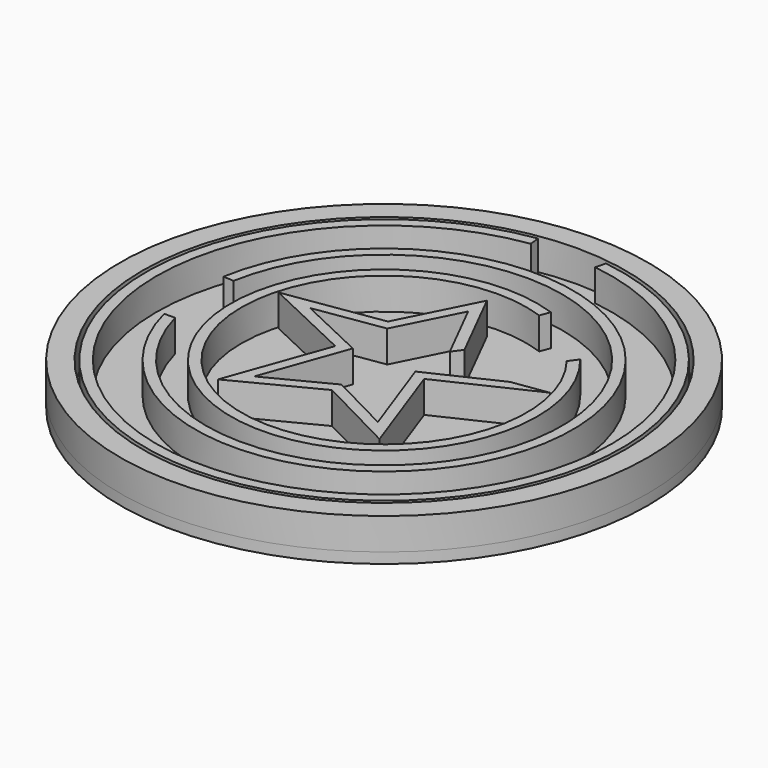
from build123d import *

# Parameters (mm, degrees)
F0_R     = 50
F0_R_2   = 45.8000004292
F1_DEPTH = 2
F2_DEPTH = 6
F3_DEPTH = 6


# Not quite as in the source:
# - a feature names something its author has since deleted; it is built from what else it names


with BuildPart() as f1:
    # F0 (on Top) → F1 (new body)
    with BuildSketch(Plane.XY):
        Circle(F0_R)
        Circle(F0_R_2, mode=Mode.SUBTRACT)
        Circle(F0_R_2)
        with BuildLine():
            ThreePointArc((6.3153904824, 44.6486646761), (0.1018848259, -45.0929820902), (-6.5170868077, 44.6196704811))
            Line((-6.5170868077, 44.6196704811), (-6.3065913026, 42.6291207003))
            ThreePointArc((-6.3065913026, 42.6291207003), (0.2401945365, -43.0924277817), (5.83099002, 42.6967748305))
            Line((5.83099002, 42.6967748305), (6.3153904824, 44.6486646761))
        make_face(mode=Mode.SUBTRACT)
        with BuildLine():
            ThreePointArc((22.5482578893, 18.2677764277), (-16.757499251, -23.6922309693), (9.7139592016, 27.3454673773))
            Line((9.7139592016, 27.3454673773), (9.0060023348, 25.4744817671))
            ThreePointArc((9.0060023348, 25.4744817671), (-15.8011926323, -21.9175639786), (21.3231605276, 16.5945811779))
            Line((21.3231605276, 16.5945811779), (22.5482578893, 18.2677764277))
        make_face(mode=Mode.SUBTRACT)
        with BuildLine():
            ThreePointArc((-35.229941381, 6.0022501649), (35.7099355205, 1.405802927), (-34.6490596367, -8.7531961618))
            Line((-34.6490596367, -8.7531961618), (-32.5798660552, -8.7622896596))
            ThreePointArc((-32.5798660552, -8.7622896596), (33.7056090039, 1.4687797411), (-33.2185830072, 5.8950093511))
            Line((-33.2185830072, 5.8950093511), (-35.229941381, 6.0022501649))
        make_face(mode=Mode.SUBTRACT)
        Polygon((5.925275698, 8.1554423446), (0, 19.9105534703), (-5.925275698, 8.1554423446), (-18.9360616209, 6.1526993897), (-5.925275698, 0), (-11.7031296948, -16.1079761248), (0, -10.0806811245), (11.7031296948, -16.1079761248), (5.925275698, 0), (18.9360616209, 6.1526993897), (25.6938207233, 7.1360371941), (8.4203775276, -1.0324396403), (15.2991478945, -20.2096408815), (0, -12.3303402142), (-15.2991478945, -20.2096408815), (-8.4203775276, -1.0324396403), (-25.6938207233, 7.1360371941), (-7.2475921337, 9.9754547797), (0, 24.3538998118), (7.2475921337, 9.9754547797), align=None, mode=Mode.SUBTRACT)
        with BuildLine():
            Line((-6.3065913026, 42.6291207003), (-6.5170868077, 44.6196704811))
            ThreePointArc((-6.5170868077, 44.6196704811), (0.1018848259, -45.0929820902), (6.3153904824, 44.6486646761))
            Line((6.3153904824, 44.6486646761), (5.83099002, 42.6967748305))
            ThreePointArc((5.83099002, 42.6967748305), (0.2401945365, -43.0924277817), (-6.3065913026, 42.6291207003))
        make_face()
        with BuildLine():
            Line((-32.5798660552, -8.7622896596), (-34.6490596367, -8.7531961618))
            ThreePointArc((-34.6490596367, -8.7531961618), (35.7099355205, 1.405802927), (-35.229941381, 6.0022501649))
            Line((-35.229941381, 6.0022501649), (-33.2185830072, 5.8950093511))
            ThreePointArc((-33.2185830072, 5.8950093511), (33.7056090039, 1.4687797411), (-32.5798660552, -8.7622896596))
        make_face()
        with BuildLine():
            Line((9.0060023348, 25.4744817671), (9.7139592016, 27.3454673773))
            ThreePointArc((9.7139592016, 27.3454673773), (-16.757499251, -23.6922309693), (22.5482578893, 18.2677764277))
            Line((22.5482578893, 18.2677764277), (21.3231605276, 16.5945811779))
            ThreePointArc((21.3231605276, 16.5945811779), (-15.8011926323, -21.9175639786), (9.0060023348, 25.4744817671))
        make_face()
        Polygon((-5.925275698, 8.1554423446), (0, 19.9105534703), (5.925275698, 8.1554423446), (7.2475921337, 9.9754547797), (0, 24.3538998118), (-7.2475921337, 9.9754547797), (-25.6938207233, 7.1360371941), (-8.4203775276, -1.0324396403), (-15.2991478945, -20.2096408815), (0, -12.3303402142), (15.2991478945, -20.2096408815), (8.4203775276, -1.0324396403), (25.6938207233, 7.1360371941), (18.9360616209, 6.1526993897), (5.925275698, 0), (11.7031296948, -16.1079761248), (0, -10.0806811245), (-11.7031296948, -16.1079761248), (-5.925275698, 0), (-18.9360616209, 6.1526993897), align=None)
    extrude(amount=-F1_DEPTH)

    # F0 (on Top) → F2 (join)
    with BuildSketch(Plane.XY):
        with BuildLine():
            Line((-6.3065913026, 42.6291207003), (-6.5170868077, 44.6196704811))
            ThreePointArc((-6.5170868077, 44.6196704811), (0.1018848259, -45.0929820902), (6.3153904824, 44.6486646761))
            Line((6.3153904824, 44.6486646761), (5.83099002, 42.6967748305))
            ThreePointArc((5.83099002, 42.6967748305), (0.2401945365, -43.0924277817), (-6.3065913026, 42.6291207003))
        make_face()
        with BuildLine():
            Line((9.0060023348, 25.4744817671), (9.7139592016, 27.3454673773))
            ThreePointArc((9.7139592016, 27.3454673773), (-16.757499251, -23.6922309693), (22.5482578893, 18.2677764277))
            Line((22.5482578893, 18.2677764277), (21.3231605276, 16.5945811779))
            ThreePointArc((21.3231605276, 16.5945811779), (-15.8011926323, -21.9175639786), (9.0060023348, 25.4744817671))
        make_face()
        with BuildLine():
            Line((-32.5798660552, -8.7622896596), (-34.6490596367, -8.7531961618))
            ThreePointArc((-34.6490596367, -8.7531961618), (35.7099355205, 1.405802927), (-35.229941381, 6.0022501649))
            Line((-35.229941381, 6.0022501649), (-33.2185830072, 5.8950093511))
            ThreePointArc((-33.2185830072, 5.8950093511), (33.7056090039, 1.4687797411), (-32.5798660552, -8.7622896596))
        make_face()
        Polygon((-5.925275698, 8.1554423446), (0, 19.9105534703), (5.925275698, 8.1554423446), (7.2475921337, 9.9754547797), (0, 24.3538998118), (-7.2475921337, 9.9754547797), (-25.6938207233, 7.1360371941), (-8.4203775276, -1.0324396403), (-15.2991478945, -20.2096408815), (0, -12.3303402142), (15.2991478945, -20.2096408815), (8.4203775276, -1.0324396403), (25.6938207233, 7.1360371941), (18.9360616209, 6.1526993897), (5.925275698, 0), (11.7031296948, -16.1079761248), (0, -10.0806811245), (-11.7031296948, -16.1079761248), (-5.925275698, 0), (-18.9360616209, 6.1526993897), align=None)
    extrude(amount=F2_DEPTH)


with BuildPart() as f3:
    # F0 (on Top) → F3 (new body)
    with BuildSketch(Plane.XY):
        Circle(F0_R)
        Circle(F0_R_2, mode=Mode.SUBTRACT)
    extrude(amount=F3_DEPTH)


solid = Compound([f1.part, f3.part])
